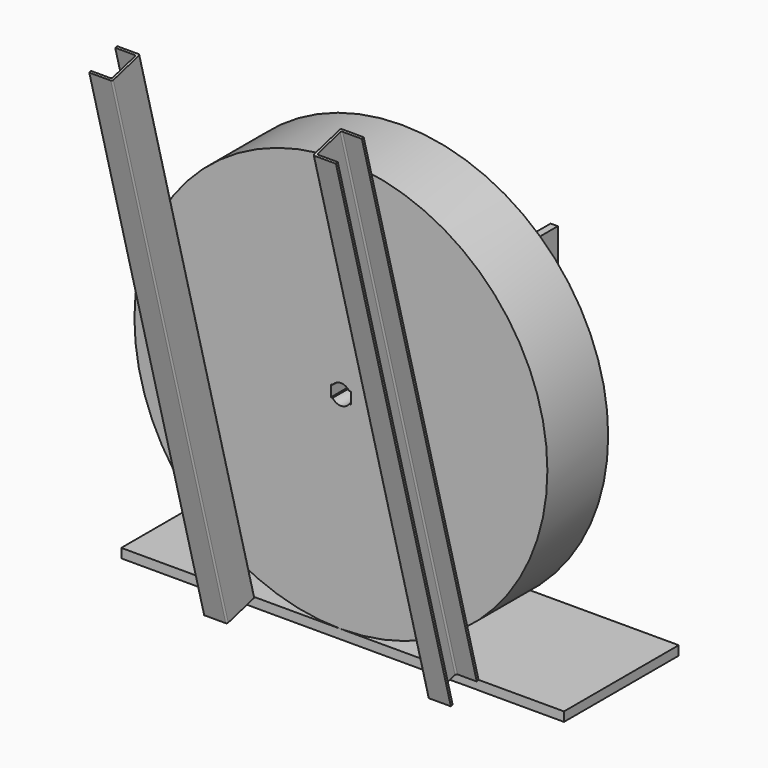
from build123d import *

# Parameters (mm, degrees)
F0_R      = 720
F0_R_2    = 35
F1_DEPTH  = 265
F3_DEPTH  = 265.001
F4_W      = 1543.660223484
F4_H      = 32.3074746132
F5_DEPTH  = 500
F7_START  = -300
F7_DEPTH  = 80
F8_START  = 400
F8_DEPTH  = 80
F9_W      = 72
F9_H      = 109
F10_DEPTH = 2095.9054427361
F11_R     = 5
F11_2_R   = 5
F12_R     = 5
F13_R     = 5
F14_R     = 5
F15_R     = 5
F17_DEPTH = 25


# Not quite as in the source:
# - a feature names something its author has since deleted; it is built from what else it names


with BuildPart() as f1:
    # F0 (on Front) → F1 (new body)
    with BuildSketch(Plane.XZ):
        Circle(F0_R)
        Circle(F0_R_2, mode=Mode.SUBTRACT)
    extrude(amount=F1_DEPTH)

    # F2 (on face) → F3 (cut, through all)
    with BuildSketch(Plane.XZ.offset(265)):
        with BuildLine():
            ThreePointArc((28.7228132327, 20), (33.3938502059, 10.4809717311), (35, 0))
            Line((35, 0), (35, 20))
            Line((35, 20), (28.7228132327, 20))
        make_face()
        with BuildLine():
            Line((35, -20), (35, 0))
            ThreePointArc((35, 0), (33.3938502059, -10.4809717311), (28.7228132327, -20))
            Line((28.7228132327, -20), (35, -20))
        make_face()
        with BuildLine():
            ThreePointArc((-28.7228132327, -20), (-33.3938502035, -10.4809717386), (-35, -1.57e-08))
            Line((-35, -1.57e-08), (-35, -20))
            Line((-35, -20), (-28.7228132327, -20))
        make_face()
        with BuildLine():
            Line((-35, 20), (-35, -1.57e-08))
            ThreePointArc((-35, -1.57e-08), (-33.3938502082, 10.4809717236), (-28.7228132327, 20))
            Line((-28.7228132327, 20), (-35, 20))
        make_face()
    extrude(amount=-F3_DEPTH, mode=Mode.SUBTRACT)


with BuildPart() as f5:
    # F4 (on face) → F5 (new body)
    with BuildSketch(Plane.XZ.offset(265)):
        with Locations((6.0311257839, -736.1537373066)):
            Rectangle(F4_W, F4_H)
    extrude(amount=-F5_DEPTH)


with BuildPart() as f7:
    # F6 (on Right) → F7 (new body)
    with BuildSketch(Plane.YZ.offset(F7_START)):
        Polygon((-385.7407282861, -752.3523806378), (-265, -720), (-765.8782422817, 1149.3030486012), (-886.6189705679, 1116.9506679634), align=None)
    extrude(amount=-F7_DEPTH)


with BuildPart() as f8:
    # F6 (on Right) → F8 (new body)
    with BuildSketch(Plane.YZ.offset(F8_START)):
        Polygon((-385.7407282861, -752.3523806378), (-265, -720), (-765.8782422817, 1149.3030486012), (-886.6189705679, 1116.9506679634), align=None)
    extrude(amount=F8_DEPTH)


with BuildPart() as f10_tool:
    # F9 (on face) → F10 (new body, through all)
    with BuildSketch(Plane(origin=(0, -338.6298762803, 1263.7839032388), x_dir=(1, 0, 0), z_dir=(0, -0.2588190451, 0.9659258263))):
        with Locations((444, -504.8200564404)):
            Rectangle(F9_W, F9_H)
        with Locations((-344, -504.8200564404)):
            Rectangle(F9_W, F9_H)
    extrude(amount=-F10_DEPTH)


with BuildPart() as f5_1:
    add(f5.part)

    # F10: cut by f10_tool
    add(f10_tool.part, mode=Mode.SUBTRACT)


with BuildPart() as f7_1:
    add(f7.part)

    # F10: cut by f10_tool
    add(f10_tool.part, mode=Mode.SUBTRACT)

    # F11
    f11_edges = [f7_1.edges().sort_by_distance(p)[0] for p in [
        (-308, -523.166528, 212.580972),
    ]]
    fillet(f11_edges, radius=F11_R)

    # F12
    f12_edges = [f7_1.edges().sort_by_distance(p)[0] for p in [
        (-300, -636.179849, 182.299144),
        (-300, -515.439121, 214.651524),
    ]]
    fillet(f12_edges, radius=F12_R)

    # F13
    f13_edges = [f7_1.edges().sort_by_distance(p)[0] for p in [
        (-308, -628.452443, 184.369696),
    ]]
    fillet(f13_edges, radius=F13_R)


with BuildPart() as f8_1:
    add(f8.part)

    # F10: cut by f10_tool
    add(f10_tool.part, mode=Mode.SUBTRACT)

    # F11#2
    f11_2_edges = [f8_1.edges().sort_by_distance(p)[0] for p in [
        (400, -515.439121, 214.651524),
        (400, -636.179849, 182.299144),
    ]]
    fillet(f11_2_edges, radius=F11_2_R)

    # F14
    f14_edges = [f8_1.edges().sort_by_distance(p)[0] for p in [
        (408, -523.166528, 212.580972),
    ]]
    fillet(f14_edges, radius=F14_R)

    # F15
    f15_edges = [f8_1.edges().sort_by_distance(p)[0] for p in [
        (408, -628.452443, 184.369696),
    ]]
    fillet(f15_edges, radius=F15_R)


with BuildPart() as f17:
    # F16 (on Right) → F17 (new body)
    with BuildSketch(Plane.YZ):
        Polygon((515.1153491874, 153.0095694043), (649.089945403, -346.9904305957), (649.089945403, 153.0095694043), align=None)
    extrude(amount=F17_DEPTH)


solid = Compound([f1.part, f5_1.part, f7_1.part, f8_1.part, f17.part])
